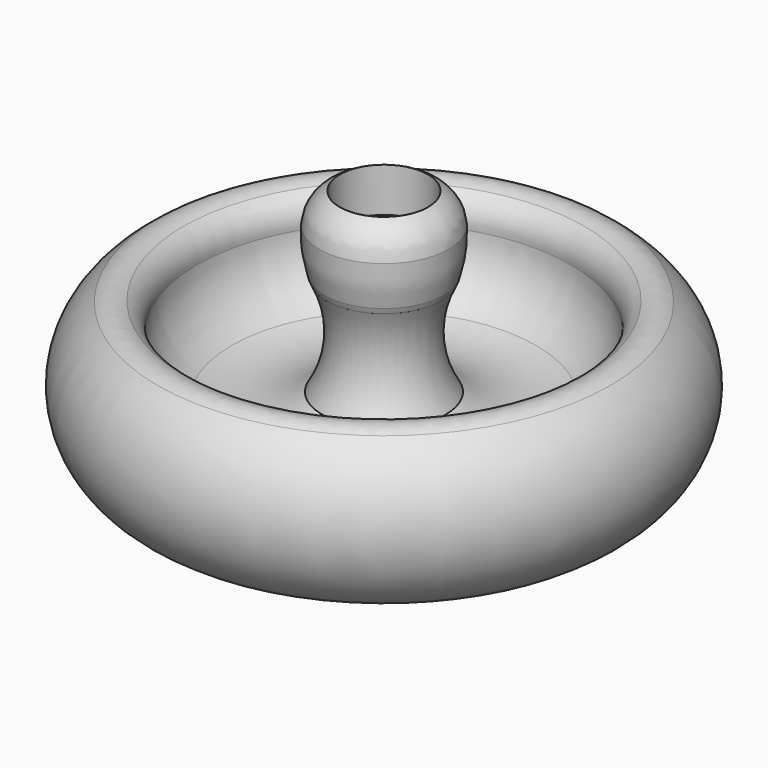
from build123d import *

# Parameters (mm, degrees)
F3_R = 5.08


# Not quite as in the source:
# - a fillet or chamfer that OpenCascade refuses, or shapes differently, is made with other operations: its cross-section is extruded or revolved along the edge and cut away or added


with BuildPart() as f1:
    # F0 (on Front) → F1 (revolve)
    with BuildSketch(Plane.XZ):
        with BuildLine():
            ThreePointArc((10.483999793, 8.704742402), (21.1854429071, 13.0945583058), (32.7157117426, 12.1757172026))
            ThreePointArc((32.7157117426, 12.1757172026), (39.3120301411, 9.7731057066), (46.3185813438, 9.3347010317))
            ThreePointArc((46.3185813438, 9.3347010317), (56.913275672, 26.1384147265), (47.1934687719, 43.4628972777))
            ThreePointArc((47.1934687719, 43.4628972777), (41.9646383543, 41.683671942), (40.3277240694, 36.4085584879))
            ThreePointArc((40.3277240694, 36.4085584879), (38.2986433941, 28.968598665), (32.7733010054, 23.5889367759))
            ThreePointArc((32.7733010054, 23.5889367759), (22.8030292444, 21.94298724), (13.3149474859, 25.4203099757))
            ThreePointArc((13.3149474859, 25.4203099757), (10.0580612498, 36.2038345129), (12.6281818375, 47.1713405905))
            ThreePointArc((12.6281818375, 47.1713405905), (14.00678773, 55.3747288113), (12.802552498, 63.605521605))
            Line((12.802552498, 63.605521605), (9.525, 63.5605369449))
            Line((9.525, 63.5605369449), (9.525, 54.0355369449))
            Line((9.525, 54.0355369449), (0, 54.0355369449))
            Line((0, 54.0355369449), (0, 22.225))
            Line((0, 22.225), (3.175, 22.225))
            Line((3.175, 22.225), (3.175, 0.0089315357))
            add(Edge.make_bspline(
                [(3.175, 0.0089315357), (4.7820895363, 2.9935227133), (7.2318930179, 5.7395980693), (10.483999793, 8.704742402)],
                knots=[0, 0, 0, 0, 11.3595160371, 11.3595160371, 11.3595160371, 11.3595160371], degree=3))
        make_face()
        with BuildLine():
            add(Edge.make_bspline(
                [(28.9868229892, 18.1371308863), (28.9868229892, 22.7980019483), (21.1494918035, 20.4675664173), (13.3121606178, 18.1371308863), (21.1494918035, 15.8066953553), (28.9868229892, 13.4762598243), (28.9868229892, 18.1371308863)],
                knots=[0, 0, 0, 2.0943951024, 2.0943951024, 4.1887902048, 4.1887902048, 6.2831853072, 6.2831853072, 6.2831853072], degree=2, weights=[1, 0.5, 1, 0.5, 1, 0.5, 1]))
        make_face(mode=Mode.SUBTRACT)
    revolve(axis=Axis((0, 0, 38.1302684724), (0, 0, -1)))

    # F2: fillet of radius 7.62 on 3 edges, made by hand

    # F2_s1 → F2_t2 (revolve, cut)
    with BuildSketch(Plane.XZ):
        with BuildLine():
            ThreePointArc((12.3722496536, 46.678759053), (12.6421523847, 47.2778226001), (12.8594436815, 47.8979105858))
            Line((12.8594436815, 47.8979105858), (13.0053080236, 47.8537591001))
            ThreePointArc((13.0053080236, 47.8537591001), (12.8916191279, 47.4875799167), (12.7727305633, 47.1230557494))
            Line((12.7727305633, 47.1230557494), (12.762510297, 47.0993570856))
            ThreePointArc((12.762510297, 47.0993570856), (12.6338808137, 46.8556010296), (12.5083701151, 46.6102245366))
            Line((12.5083701151, 46.6102245366), (12.3722496536, 46.678759053))
        make_face()
    revolve(axis=Axis((0, 0, 47.1713405905), (0, 0, -1)), mode=Mode.SUBTRACT)

    # F2_s3 → F2_t4 (revolve, cut)
    with BuildSketch(Plane.XZ):
        with BuildLine():
            ThreePointArc((13.9741009654, 57.0120678291), (12.6667334765, 60.9094464641), (9.525, 63.5605369449))
            Line((9.525, 63.5605369449), (9.5882234526, 63.6992040103))
            ThreePointArc((9.5882234526, 63.6992040103), (11.1616847443, 63.7354149226), (12.8004609933, 63.7579072526))
            Line((12.8004609933, 63.7579072526), (12.9480931941, 63.6507285267))
            ThreePointArc((12.9480931941, 63.6507285267), (13.7452153435, 60.372207963), (14.1263064373, 57.0197655122))
            Line((14.1263064373, 57.0197655122), (13.9741009654, 57.0120678291))
        make_face()
    revolve(axis=Axis((0, 0, 63.605521605), (0, 0, -1)), mode=Mode.SUBTRACT)

    # F3
    f3_edges = [f1.edges().sort_by_distance(p)[0] for p in [
        (-47.193469, 0, 43.462897),
        (-46.318581, 0, 9.334701),
        (56.913276, 0, 26.138415),
    ]]
    fillet(f3_edges, radius=F3_R)


solid = f1.part
